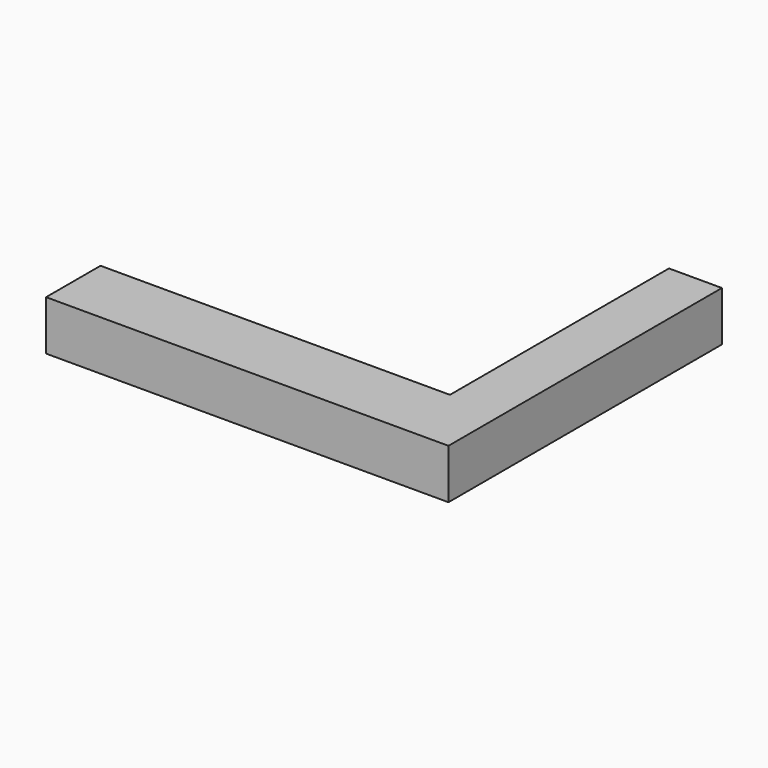
from build123d import *

# Parameters (mm, degrees)
F0_W     = 39.360307157
F0_H     = 36.9374714792
F1_DEPTH = 254
F2_W     = 50.564668417
F2_H     = 36.9374714792
F3_DEPTH = 259.6821213


# Not quite as in the source:
# - an extrude ends at something that could not be found from the text; its depth is read off the source's solid


with BuildPart() as f1:
    # F0 (on Front) → F1 (new body)
    with BuildSketch(Plane.XZ):
        with Locations((19.6801535785, 18.4687357396)):
            Rectangle(F0_W, F0_H)
    extrude(amount=F1_DEPTH)

    # F2 (on face) → F3 (join, through all)
    with BuildSketch(Plane(origin=(0, 0, 0), x_dir=(0, -1, 0), z_dir=(-1, 0, 0))):
        with Locations((228.7176657915, 18.4687357396)):
            Rectangle(F2_W, F2_H)
    extrude(amount=F3_DEPTH)


solid = f1.part
